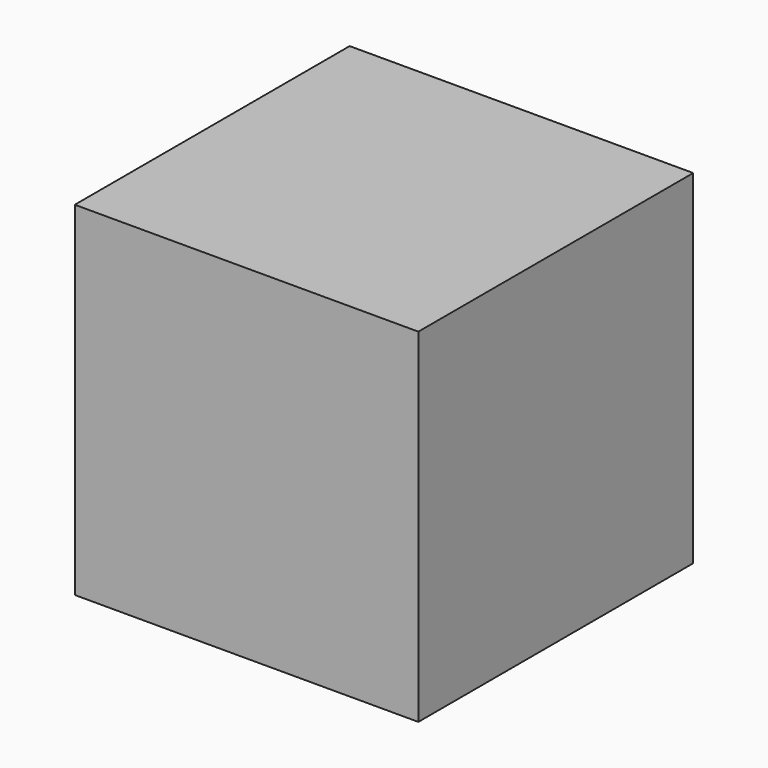
from build123d import *

# Parameters (mm, degrees)
F1_W     = 101.6
F1_H     = 101.6
F2_DEPTH = 50.8


# Not quite as in the source:
# - a variable given as a bare number and used for a length is read in inches; the dataset says mm whatever the document's units were


with BuildPart() as f2:
    # F1 (on Top) → F2 (new body, symmetric)
    with BuildSketch(Plane.XY):
        Rectangle(F1_W, F1_H)
    extrude(amount=F2_DEPTH, both=True)


solid = f2.part
